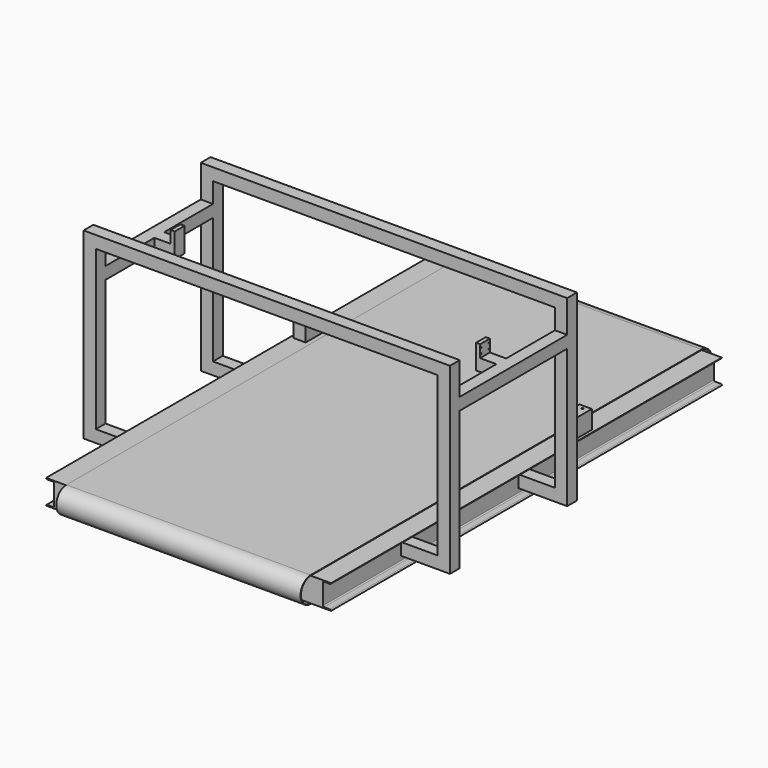
from build123d import *

# Parameters (mm, degrees)
F1_DEPTH  = 762
F3_DEPTH  = 1524
F4_R      = 6.34999
F5_W      = 76.2
F5_H      = 152.4
F5_R      = 5.55625
F6_DEPTH  = 114.3
F8_DEPTH  = 76.2
F11_DEPTH = 76.2
F13_D     = 5.1054
F13_DEPTH = 16.51
F13_TIP   = 1.5338169022
F14_W     = 76.2
F14_H     = 76.2
F15_DEPTH = 838.2
F16_W     = 127
F16_H     = 76.2
F17_DEPTH = 76.2
F18_W     = 25.4
F18_H     = 76.2
F19_DEPTH = 76.2
F21_D     = 5.1054
F21_DEPTH = 16.51
F21_TIP   = 1.5338169022


# Not quite as in the source:
# - a fillet or chamfer is up to 0.001 mm smaller than in the source, because OpenCascade refuses the exact size


with BuildPart() as f1:
    # F0 (on Right) → F1 (new body, symmetric)
    with BuildSketch(Plane.YZ):
        with BuildLine():
            ThreePointArc((1524, -157.1625), (1603.375, -77.7875), (1524, 1.5875))
            Line((1524, 1.5875), (-1524, 1.5875))
            ThreePointArc((-1524, 1.5875), (-1603.375, -77.7875), (-1524, -157.1625))
            Line((-1524, -157.1625), (1524, -157.1625))
        make_face()
        with BuildLine():
            Line((-1524, -1.5875), (1524, -1.5875))
            ThreePointArc((1524, -1.5875), (1600.2, -77.7875), (1524, -153.9875))
            Line((1524, -153.9875), (-1524, -153.9875))
            ThreePointArc((-1524, -153.9875), (-1600.2, -77.7875), (-1524, -1.5875))
        make_face(mode=Mode.SUBTRACT)
    extrude(amount=F1_DEPTH, both=True)


with BuildPart() as f3:
    # F2 (on Front) → F3 (new body, symmetric)
    with BuildSketch(Plane.XZ):
        Polygon((-889, -153.9875), (889, -153.9875), (889, -147.6375), (838.2, -147.6375), (838.2, -7.9375), (889, -7.9375), (889, -1.5875), (-889, -1.5875), (-889, -7.9375), (-838.2, -7.9375), (-838.2, -147.6375), (-889, -147.6375), align=None)
    extrude(amount=F3_DEPTH, both=True)

    # F4 (radius 6.35 in the source; OpenCascade refuses exactly that, so slightly less here)
    f4_edges = [f3.edges().sort_by_distance(p)[0] for p in [
        (-889, 0, -7.9375),
        (-838.2, 0, -7.9375),
        (-838.2, 0, -147.6375),
        (-889, 0, -147.6375),
        (889, 0, -7.9375),
        (838.2, 0, -147.6375),
        (889, 0, -147.6375),
        (838.2, 0, -7.9375),
    ]]
    fillet(f4_edges, radius=F4_R)

    # F5 (on face) → F6 (join)
    with BuildSketch(Plane.XY.offset(-1.5875)):
        with Locations((831.85, 457.2)):
            Rectangle(F5_W, F5_H)
        with Locations((831.85, 406.4)):
            Circle(F5_R, mode=Mode.SUBTRACT)
        with Locations((831.85, 508)):
            Circle(F5_R, mode=Mode.SUBTRACT)
        with Locations((-831.85, 457.2)):
            Rectangle(F5_W, F5_H)
        with Locations((-831.85, 406.4)):
            Circle(F5_R, mode=Mode.SUBTRACT)
        with Locations((-831.85, 508)):
            Circle(F5_R, mode=Mode.SUBTRACT)
    extrude(amount=F6_DEPTH)

    # F7 (on Front) → F8 (join)
    with BuildSketch(Plane.XZ):
        Polygon((1066.8, -39.6875), (838.2, -39.6875), (838.2, -115.8875), (1143, -115.8875), (1143, 1027.1125), (-1143, 1027.1125), (-1143, -115.8875), (-838.2, -115.8875), (-838.2, -39.6875), (-1066.8, -39.6875), (-1066.8, 950.9125), (1066.8, 950.9125), align=None)
    extrude(amount=-F8_DEPTH)

    # F10 (on offset) → F11 (join)
    with BuildSketch(Plane.XZ.offset(914.4)):
        Polygon((1066.8, -39.6875), (838.2, -39.6875), (838.2, -115.8875), (1143, -115.8875), (1143, 1027.1125), (-1143, 1027.1125), (-1143, -115.8875), (-838.2, -115.8875), (-838.2, -39.6875), (-1066.8, -39.6875), (-1066.8, 950.9125), (1066.8, 950.9125), align=None)
    extrude(amount=-F11_DEPTH)

    # F13 (one way)
    with BuildSketch(Plane(origin=(0, 0, 950.9125), x_dir=(1, 0, 0), z_dir=(0, 0, -1))):
        with Locations((-952.5, -19.05), (-952.5, -57.15), (-800.1, -19.05), (-800.1, -57.15), (-647.7, -57.15), (-647.7, -19.05), (647.7, -57.15), (647.7, -19.05), (800.1, -57.15), (800.1, -19.05), (952.5, -19.05), (952.5, -57.15), (-952.5, 857.25), (-952.5, 895.35), (-800.1, 895.35), (-800.1, 857.25), (-647.7, 857.25), (-647.7, 895.35), (647.7, 895.35), (647.7, 857.25), (800.1, 857.25), (800.1, 895.35), (952.5, 895.35), (952.5, 857.25)):
            Circle(F13_D / 2)
    extrude(amount=-F13_DEPTH, mode=Mode.SUBTRACT)
    with Locations(Plane(origin=(0, 0, 950.9125), x_dir=(1, 0, 0), z_dir=(0, 0, -1))):
        with Locations((-952.5, -19.05), (-952.5, -57.15), (-800.1, -19.05), (-800.1, -57.15), (-647.7, -57.15), (-647.7, -19.05), (647.7, -57.15), (647.7, -19.05), (800.1, -57.15), (800.1, -19.05), (952.5, -19.05), (952.5, -57.15), (-952.5, 857.25), (-952.5, 895.35), (-800.1, 895.35), (-800.1, 857.25), (-647.7, 857.25), (-647.7, 895.35), (647.7, 895.35), (647.7, 857.25), (800.1, 857.25), (800.1, 895.35), (952.5, 895.35), (952.5, 857.25)):
            with Locations((0, 0, -(F13_DEPTH + F13_TIP / 2))):  # 118° drill point
                Cone(0, F13_D / 2, F13_TIP, mode=Mode.SUBTRACT)

    # F14 (on face) → F15 (join, through all)
    with BuildSketch(Plane.XZ):
        with Locations((1104.9, 787.4127)):
            Rectangle(F14_W, F14_H)
    extrude(amount=F15_DEPTH)

    # F16 (on face) → F17 (join, through all)
    with BuildSketch(Plane.XY.offset(825.5127)):
        with Locations((1003.3, -419.1)):
            Rectangle(F16_W, F16_H)
    extrude(amount=-F17_DEPTH)

    # F18 (on face) → F19 (join)
    with BuildSketch(Plane.XY.offset(825.5127)):
        with Locations((952.5, -419.1)):
            Rectangle(F18_W, F18_H)
    extrude(amount=F19_DEPTH)

    # F21
    with Locations(Plane.YZ.offset(965.2)):
        with Locations((-448.46875, 879.8814), (-448.46875, 847.344), (-389.73125, 847.344), (-389.73125, 879.8814)):
            Hole(F21_D / 2, depth=F21_DEPTH)
            with Locations((0, 0, -(F21_DEPTH + F21_TIP / 2))):  # 118° drill point
                Cone(0, F21_D / 2, F21_TIP, mode=Mode.SUBTRACT)

    # F22: F3 across plane


with BuildPart() as f3_1:
    add(f3.part)
    add(f3.part.mirror(Plane.YZ))


solid = Compound([f1.part, f3_1.part])
